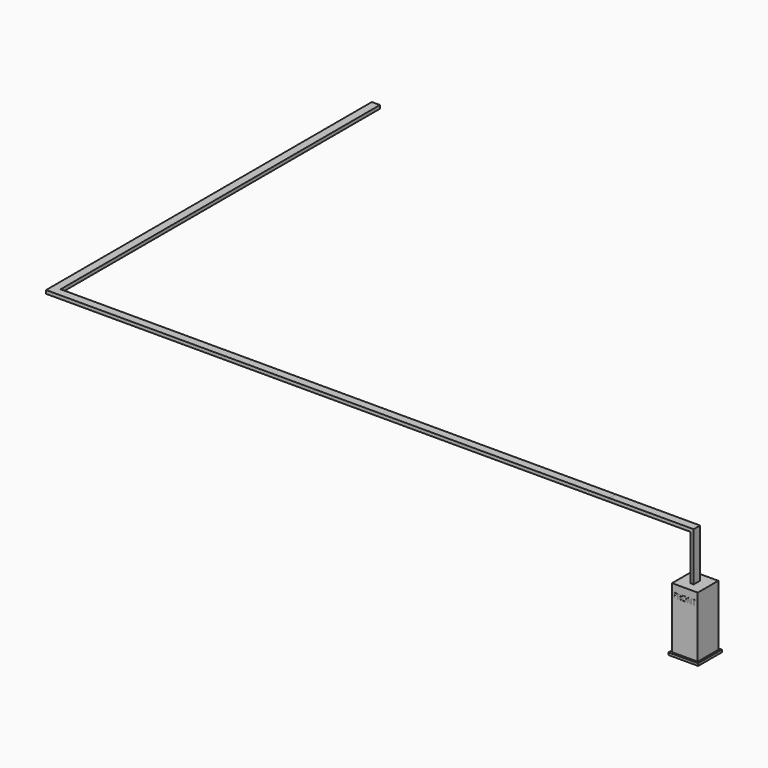
from build123d import *

# Parameters (mm, degrees)
F0_W         = 1117.6
F0_H         = 1117.6
F1_DEPTH     = 88.9
F2_W         = 965.2
F2_H         = 965.2
F3_DEPTH     = 2286
F4_TEXT_SIZE = 265.7112148073
F5_DEPTH     = 2.54
F6_TEXT_SIZE = 381.0172279676
F7_DEPTH     = 2.54
F8_W         = 127
F8_H         = 304.8
F9_DEPTH     = 1828.8
F10_W        = 304.8
F10_H        = 127
F11_DEPTH    = 3048
F12_DEPTH    = 67056
F13_DEPTH    = 45872.4
F14_W        = 304.8
F14_H        = 127
F15_DEPTH    = 15011.4


# Not quite as in the source:
# - Text() gives the source's letters only with a copy of the font that has no kerning and outlines rounded to 1/6400 em; it was checked with that copy


with BuildPart() as f1:
    # F0 (on Top) → F1 (new body)
    with BuildSketch(Plane.XY):
        with Locations((558.8, 558.8)):
            Rectangle(F0_W, F0_H)
    extrude(amount=F1_DEPTH)

    # F2 (on face) → F3 (join)
    with BuildSketch(Plane.XY.offset(88.9)):
        with Locations((558.8, 558.8)):
            Rectangle(F2_W, F2_H)
    extrude(amount=F3_DEPTH)

    # F4 (on face) → F5 (join)
    with BuildSketch(Plane.XZ.offset(-76.2)):
        with Locations((120.2508807182, 1906.7323207855)):
            Text('FRONT', F4_TEXT_SIZE, font='Open Sans', text_align=(TextAlign.LEFT, TextAlign.BOTTOM))
    extrude(amount=F5_DEPTH)

    # F6 (on face) → F7 (join)
    with BuildSketch(Plane(origin=(0, 1041.4, 0), x_dir=(-1, 0, 0), z_dir=(0, 1, 0))):
        with Locations((-1063.1536883198, 1848.6394882202)):
            Text('BACK', F6_TEXT_SIZE, font='Open Sans', text_align=(TextAlign.LEFT, TextAlign.BOTTOM))
    extrude(amount=F7_DEPTH)

    # F8 (on face) → F9 (join)
    with BuildSketch(Plane.XY.offset(2374.9)):
        with Locations((558.8, 558.8)):
            Rectangle(F8_W, F8_H)
    extrude(amount=F9_DEPTH)

    # F10 (on face) → F11 (join)
    with BuildSketch(Plane(origin=(495.3, 0, 0), x_dir=(0, -1, 0), z_dir=(-1, 0, 0))):
        with Locations((-558.8, 4140.2)):
            Rectangle(F10_W, F10_H)
    extrude(amount=F11_DEPTH)


with BuildPart() as f12:
    # F12 (new): a face of the model
    f12_faces = [f1.part.faces().sort_by_distance(p)[0] for p in [
        (-2552.7, 558.8, 4140.2),
    ]]
    extrude(f12_faces, amount=F12_DEPTH)

    # F13 (cut): a face of the model
    f13_faces = [f12.faces().sort_by_distance(p)[0] for p in [
        (-69608.7, 558.8, 4140.2),
    ]]
    extrude(f13_faces, amount=-F13_DEPTH, mode=Mode.SUBTRACT)

    # F14 (on face) → F15 (join)
    with BuildSketch(Plane(origin=(0, 711.2, 0), x_dir=(-1, 0, 0), z_dir=(0, 1, 0))):
        with Locations((23583.9, 4140.2)):
            Rectangle(F14_W, F14_H)
    extrude(amount=F15_DEPTH)


solid = Compound([f1.part, f12.part])
